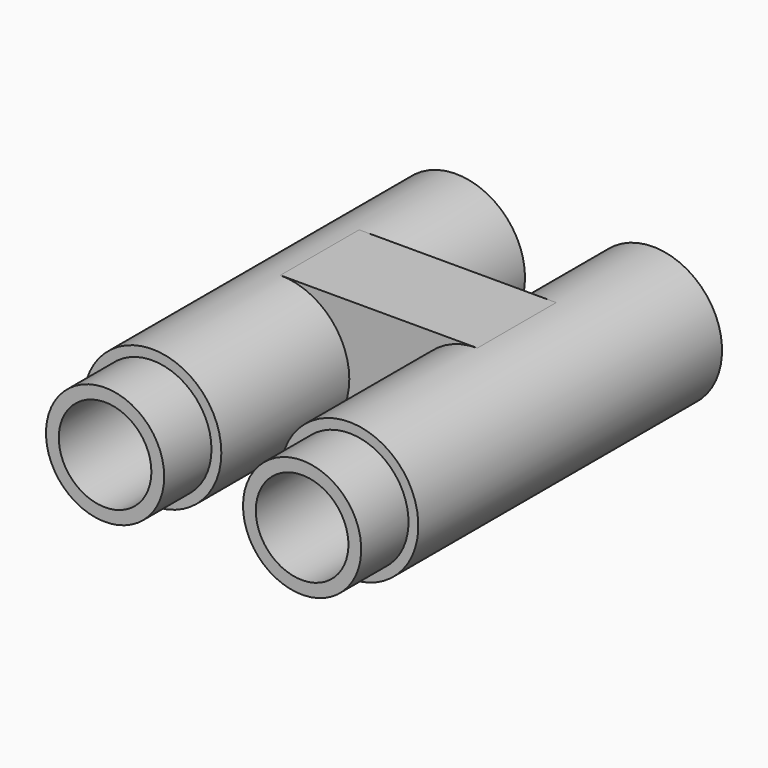
from build123d import *

# Parameters (mm, degrees)
F1_R          = 8.89
F1_R_2        = 5.969
F3_R          = 8.89
F3_R_2        = 7.62
F4_DEPTH      = 7.62
F5_DEPTH      = 25.4
F5_DEPTH_BACK = 25.4
F6_R          = 7.62
F7_R          = 7.62
F8_DEPTH      = 38.1
F0_W          = 25.4
F0_H          = 12.7
F9_DEPTH      = 8.89
F9_DEPTH_BACK = 8.89
F10_DEPTH     = 25.4
F11_DEPTH     = 38.1


with BuildPart() as f2:
    # F2: sweep along a path in F0
    with BuildLine(Plane.XY) as f2_path:
        Line((0, 0), (0, 124.469906))
        ThreePointArc((0, 124.469906), (12.7, 137.169906), (25.4, 124.469906))
        Line((25.4, 124.469906), (25.4, 0))
    # F1 (on Front) → F2 (sweep)
    with BuildSketch(Plane.XZ):
        Circle(F1_R)
        Circle(F1_R_2, mode=Mode.SUBTRACT)
    sweep(path=f2_path.line)

    # F3 (on face) → F4 (cut)
    with BuildSketch(Plane.XZ):
        Circle(F3_R)
        Circle(F3_R_2, mode=Mode.SUBTRACT)
        with BuildLine():
            ThreePointArc((34.29, 0), (25.4, 8.89), (16.51, 0))
            ThreePointArc((16.51, 0), (25.4, -8.89), (34.29, 0))
        make_face()
        with BuildLine():
            ThreePointArc((33.02, 0), (25.4, -7.62), (17.78, 0))
            ThreePointArc((17.78, 0), (25.4, 7.62), (33.02, 0))
        make_face(mode=Mode.SUBTRACT)
    extrude(amount=-F4_DEPTH, mode=Mode.SUBTRACT)

    # F0 (on Top) → F5 (cut, two sides)
    with BuildSketch(Plane.XY) as f5_sk:
        with BuildLine():
            Line((-27.3511596024, 56.5561708785), (0, 56.5561708785))
            Line((0, 56.5561708785), (0, 124.469906))
            ThreePointArc((0, 124.469906), (3.7197438789, 133.4501621211), (12.7, 137.169906))
            ThreePointArc((12.7, 137.169906), (21.6802561211, 133.4501621211), (25.4, 124.469906))
            Line((25.4, 124.469906), (25.4, 56.5561708785))
            Line((25.4, 56.5561708785), (45.1116599143, 56.5561708785))
            Line((45.1116599143, 56.5561708785), (45.1116599143, 146.6434597969))
            Line((45.1116599143, 146.6434597969), (-27.3511596024, 146.6434597969))
            Line((-27.3511596024, 146.6434597969), (-27.3511596024, 56.5561708785))
        make_face()
        with BuildLine():
            Line((0, 124.469906), (0, 56.5561708785))
            Line((0, 56.5561708785), (12.7, 56.5561708785))
            Line((12.7, 56.5561708785), (12.7, 137.169906))
            ThreePointArc((12.7, 137.169906), (3.7197438789, 133.4501621211), (0, 124.469906))
        make_face()
        with BuildLine():
            Line((12.7, 56.5561708785), (25.4, 56.5561708785))
            Line((25.4, 56.5561708785), (25.4, 124.469906))
            ThreePointArc((25.4, 124.469906), (21.6802561211, 133.4501621211), (12.7, 137.169906))
            Line((12.7, 137.169906), (12.7, 56.5561708785))
        make_face()
    extrude(amount=-F5_DEPTH, mode=Mode.SUBTRACT)
    extrude(f5_sk.sketch, amount=F5_DEPTH_BACK, mode=Mode.SUBTRACT)

    # F6 (on face) + F7 (on face) → F8 (cut)
    with BuildSketch(Plane(origin=(0, 56.5561708785, 0), x_dir=(-1, 0, 0), z_dir=(0, 1, 0))):
        with Locations((-25.4, 0)):
            Circle(F6_R)
    with BuildSketch(Plane(origin=(0, 56.5561708785, 0), x_dir=(-1, 0, 0), z_dir=(0, 1, 0))):
        Circle(F7_R)
    extrude(amount=-F8_DEPTH, mode=Mode.SUBTRACT)

    # F0 (on Top) → F9 (join, two sides)
    with BuildSketch(Plane.XY) as f9_sk:
        with Locations((12.7, 34.5915263355)):
            Rectangle(F0_W, F0_H)
    extrude(amount=F9_DEPTH)
    extrude(f9_sk.sketch, amount=-F9_DEPTH_BACK)

    # F7 (on face) + F6 (on face) → F10 (cut)
    with BuildSketch(Plane(origin=(0, 56.5561708785, 0), x_dir=(-1, 0, 0), z_dir=(0, 1, 0))):
        Circle(F7_R)
    with BuildSketch(Plane(origin=(0, 56.5561708785, 0), x_dir=(-1, 0, 0), z_dir=(0, 1, 0))):
        with Locations((-25.4, 0)):
            Circle(F6_R)
    extrude(amount=-F10_DEPTH, mode=Mode.SUBTRACT)

    # F7 (on face) + F6 (on face) → F11 (cut)
    with BuildSketch(Plane(origin=(0, 56.5561708785, 0), x_dir=(-1, 0, 0), z_dir=(0, 1, 0))):
        Circle(F7_R)
    with BuildSketch(Plane(origin=(0, 56.5561708785, 0), x_dir=(-1, 0, 0), z_dir=(0, 1, 0))):
        with Locations((-25.4, 0)):
            Circle(F6_R)
    extrude(amount=-F11_DEPTH, mode=Mode.SUBTRACT)


solid = f2.part
